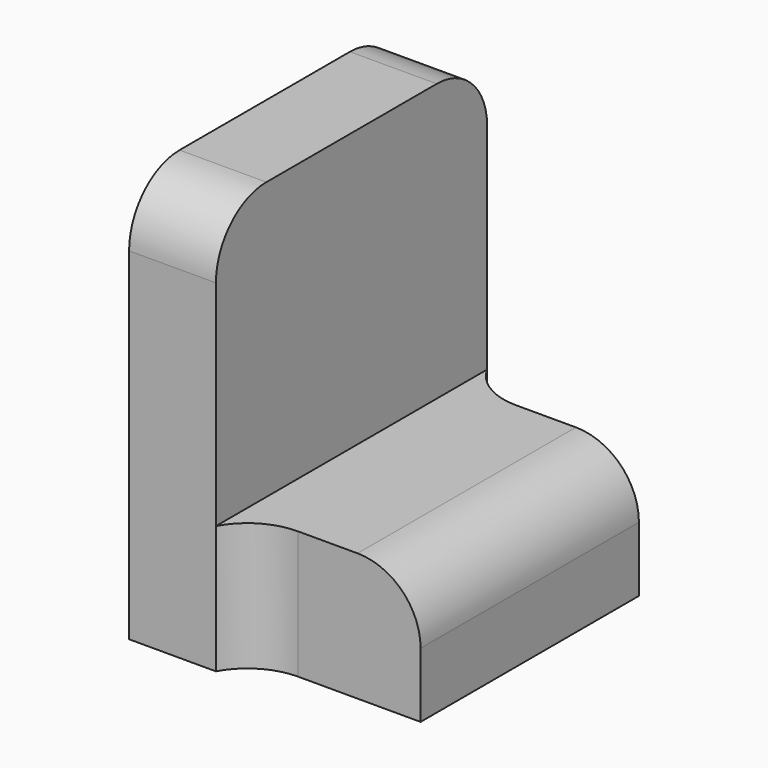
from build123d import *

# Parameters (mm, degrees)
F1_DEPTH    = 19.304
F0_W        = 4.2467024177
F0_H        = 13.0065511912
F2_DEPTH    = 6.096
F3_T1_DEPTH = 6.096
F3_T3_DEPTH = 6.096
F3_T5_DEPTH = 19.1620992743
F3_T7_DEPTH = 19.1620992743
F3_T9_DEPTH = 28.0302021899


# Not quite as in the source:
# - a fillet or chamfer that OpenCascade refuses, or shapes differently, is made with other operations: its cross-section is extruded or revolved along the edge and cut away or added


with BuildPart() as f1:
    # F0 (on Top) → F1 (new body)
    with BuildSketch(Plane.XY):
        Polygon((-6.1091380194, 8.0798277631), (-6.1091380194, 0), (-6.1091380194, -8.0798277631), (-1.9706897438, -8.0798277631), (-1.9706897438, -6.5032755956), (-1.9706897438, 6.5032755956), (-1.9706897438, 8.0798277631), align=None)
    extrude(amount=F1_DEPTH)

    # F0 (on Top) → F2 (join)
    with BuildSketch(Plane.XY):
        with Locations((0.1526614651, 0)):
            Rectangle(F0_W, F0_H)
        with Locations((4.3993638828, 0)):
            Rectangle(F0_W, F0_H)
    extrude(amount=F2_DEPTH)

    # F3: fillet of radius 3.0047301997 on 5 edges, made by hand

    # F3_s2 → F3_t1 (join)
    with BuildSketch(Plane.XY):
        with BuildLine():
            ThreePointArc((-1.9706897438, -8.0798277631), (-0.8660843797, -6.9273379324), (0.6729273014, -6.5032755956))
            Line((0.6729273014, -6.5032755956), (-1.9706897438, -6.5032755956))
            Line((-1.9706897438, -6.5032755956), (-1.9706897438, -8.0798277631))
        make_face()
    extrude(amount=F3_T1_DEPTH)

    # F3_s4 → F3_t3 (join)
    with BuildSketch(Plane.XY):
        with BuildLine():
            ThreePointArc((-1.9706897438, 8.0798277631), (-0.8660843797, 6.9273379324), (0.6729273014, 6.5032755956))
            Line((0.6729273014, 6.5032755956), (-1.9706897438, 6.5032755956))
            Line((-1.9706897438, 6.5032755956), (-1.9706897438, 8.0798277631))
        make_face()
    extrude(amount=F3_T3_DEPTH)

    # F3_s6 → F3_t5 (cut)
    with BuildSketch(Plane.YZ.offset(-13.6209635187)):
        with BuildLine():
            ThreePointArc((5.0750975634, 19.304), (7.1997626633, 18.4239349001), (8.0798277631, 16.2992698003))
            Line((8.0798277631, 16.2992698003), (8.0798277631, 19.304))
            Line((8.0798277631, 19.304), (5.0750975634, 19.304))
        make_face()
    extrude(amount=F3_T5_DEPTH, mode=Mode.SUBTRACT)

    # F3_s8 → F3_t7 (cut)
    with BuildSketch(Plane.YZ.offset(-13.6209635187)):
        with BuildLine():
            ThreePointArc((-8.0798277631, 16.2992698003), (-7.1997626633, 18.4239349001), (-5.0750975634, 19.304))
            Line((-5.0750975634, 19.304), (-8.0798277631, 19.304))
            Line((-8.0798277631, 19.304), (-8.0798277631, 16.2992698003))
        make_face()
    extrude(amount=F3_T7_DEPTH, mode=Mode.SUBTRACT)

    # F3_s10 → F3_t9 (cut)
    with BuildSketch(Plane.XZ.offset(-14.0151010949)):
        with BuildLine():
            ThreePointArc((6.5227150917, 3.0912698003), (5.6426499918, 5.2159349001), (3.517984892, 6.096))
            Line((3.517984892, 6.096), (6.5227150917, 6.096))
            Line((6.5227150917, 6.096), (6.5227150917, 3.0912698003))
        make_face()
    extrude(amount=F3_T9_DEPTH, mode=Mode.SUBTRACT)


solid = f1.part
